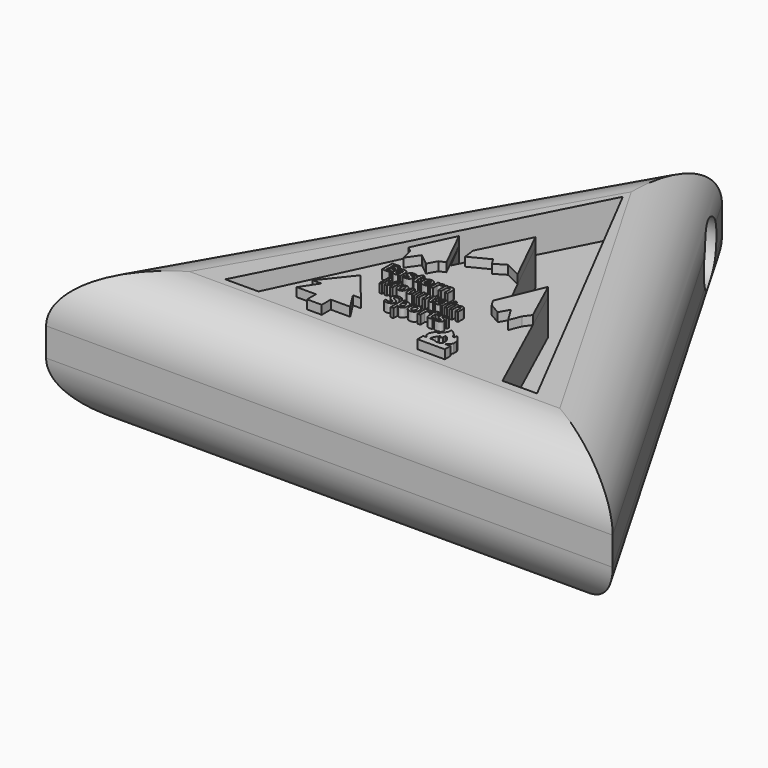
from build123d import *

# Parameters (mm, degrees)
F1_DEPTH       = 12.7
F2_R           = 5.08
F3_R           = 2.54
F4_DEPTH       = 25.4
F5_DEPTH       = 25.4
F7_DEPTH       = 3.175
F8_TEXT_SIZE   = 1.6130481122
F8_TEXT_SIZE_2 = 1.4935671869
F8_TEXT_SIZE_3 = 1.6727924554
F9_DEPTH       = 0.79375


# Not quite as in the source:
# - Text() gives the source's letters only with a copy of the font that has no kerning and outlines rounded to 1/6400 em; it was checked with that copy


with BuildPart() as f1:
    # F0 (on Top) → F1 (new body)
    with BuildSketch(Plane.XY):
        Polygon((25.4, 10.4120860291), (0, 54.4061765414), (-25.4, 10.4120860291), align=None)
    extrude(amount=F1_DEPTH)

    # F2
    f2_edges = [f1.edges().sort_by_distance(p)[0] for p in [
        (0, 10.412086, 12.7),
        (-12.7, 32.409131, 12.7),
        (12.7, 32.409131, 12.7),
        (0, 10.412086, 0),
        (-12.7, 32.409131, 0),
        (12.7, 32.409131, 0),
    ]]
    fillet(f2_edges, radius=F2_R)

    # F3 (on Right) → F4 (cut)
    with BuildSketch(Plane.YZ):
        with Locations((49.6464930475, 6.4756297506)):
            Circle(F3_R)
    extrude(amount=-F4_DEPTH, mode=Mode.SUBTRACT)

    # F3 (on Right) → F5 (cut)
    with BuildSketch(Plane.YZ):
        with Locations((49.6464930475, 6.4756297506)):
            Circle(F3_R)
    extrude(amount=F5_DEPTH, mode=Mode.SUBTRACT)

    # F6 (on face) → F7 (cut)
    with BuildSketch(Plane.XY.offset(12.7)):
        Polygon((0, 43.3048903942), (-13.9127802104, 16.1387268454), (-10.9459740387, 16.1516164506), (-4.2856149375, 30.2965939045), (-2.8930064291, 27.6344306767), (0, 33.5032902658), (4.0700379759, 25.2142827958), (5.4020984098, 28.1789656729), (10.8517583743, 16.2463190192), (13.9393955469, 16.2597335875), align=None)
    extrude(amount=-F7_DEPTH, mode=Mode.SUBTRACT)

    # F8 (on face) → F9 (join)
    with BuildSketch(Plane.XY.offset(12.7)):
        Polygon((-3.0329301953, 26.4089070261), (-2.4885963649, 26.6434270889), (-4.2856149375, 30.2965939045), (-5.9598912337, 26.7408396124), (-5.5513591506, 26.4089070261), (-5.2715335041, 25.3023244441), (-4.4956537895, 26.4089070261), (-3.4781070426, 25.5821496248), align=None)
        Polygon((-2.1321694852, 29.1778925747), (-1.9974971656, 28.1266011298), (-0.2151948459, 29.0352557385), (0.1416321466, 28.4448694438), (1.1149357306, 29.0331300348), (2.5491314526, 28.3117491111), (0, 33.5032902658), align=None)
        Polygon((5.4020984098, 28.1789656729), (3.6926330067, 24.1268407553), (4.0405294858, 23.5520545393), (5.0388406962, 22.9772701859), (5.5359300199, 23.8406371887), (6.3547962345, 22.4932394922), (6.7783221602, 23.5520545393), (7.2320062377, 24.1721755867), align=None)
        Polygon((-3.5369039979, 17.1628147364), (-4.4747111388, 18.6451561749), (-3.7637928035, 18.6451561749), (-5.9570521116, 21.3375706226), (-8.0898078158, 18.6602808535), (-7.3183854111, 18.6602808535), (-8.3166966215, 17.1476881951), (-6.592341233, 17.1476881951), (-6.592341233, 16.1516164506), (-5.2763856947, 16.1516164506), (-5.2763856947, 17.1628147364), align=None)
        Polygon((3.222388681, 16.8965011835), (3.222388681, 16.2635110319), (5.6639234535, 16.2635110319), (5.6639234535, 16.8965011835), (5.2042910829, 16.8965011835), (5.3037614562, 16.977885738), (5.5027012713, 17.1587392688), (5.5840853602, 17.3486359417), (5.5840853602, 17.4842774868), (5.5750426836, 17.7555587143), (5.457487423, 17.9544985294), (5.2314195782, 18.2529091835), (5.076367856, 18.3795075864), (5.076367856, 18.127232401), (4.942052532, 18.0539693683), (4.7250268981, 18.4518489987), (4.4356598519, 18.7050439417), (4.2186346836, 18.8316423446), (4.2186346836, 18.5332335532), (4.1101220995, 18.3071643114), (3.6941566505, 17.845986411), (3.6760712974, 18.0630125105), (3.5856440663, 18.1624814868), (3.5766013898, 18.0358830839), (3.2872343436, 17.520448193), (3.2872343436, 17.2039531171), (3.5223450977, 16.8965011835), align=None)
        Polygon((4.1632531211, 16.8965011835), (3.8513967302, 16.8965011835), (3.8513967302, 17.1218030155), (3.9696870372, 17.3368752003), (4.1094846092, 17.5089351833), (4.1094846092, 17.6809933037), (4.2385286652, 17.6164712757), (4.2385286652, 17.3906441778), (4.4320947491, 17.6164712757), (4.4320947491, 17.9068204015), (4.6686753631, 17.7670214325), (4.8407344148, 17.5304412842), (4.969778005, 17.3368752003), (4.969778005, 17.1325560659), (4.969778005, 16.8965011835), (4.8447887201, 16.7942375955), (4.464355763, 16.7776849121), align=None, mode=Mode.SUBTRACT)
        with Locations((-5.4803566018, 22.9911897331)):
            Text('Eastern', F8_TEXT_SIZE, font='Open Sans', font_style=FontStyle.BOLD, text_align=(TextAlign.LEFT, TextAlign.BOTTOM))
        with Locations((-4.3189604767, 21.2706010789)):
            Text('Mountain', F8_TEXT_SIZE_2, font='Open Sans', font_style=FontStyle.BOLD, text_align=(TextAlign.LEFT, TextAlign.BOTTOM))
        with Locations((-2.3402853403, 19.2919261754)):
            Text('Sports', F8_TEXT_SIZE_3, font='Open Sans', font_style=FontStyle.BOLD, text_align=(TextAlign.LEFT, TextAlign.BOTTOM))
    extrude(amount=F9_DEPTH)


solid = f1.part
